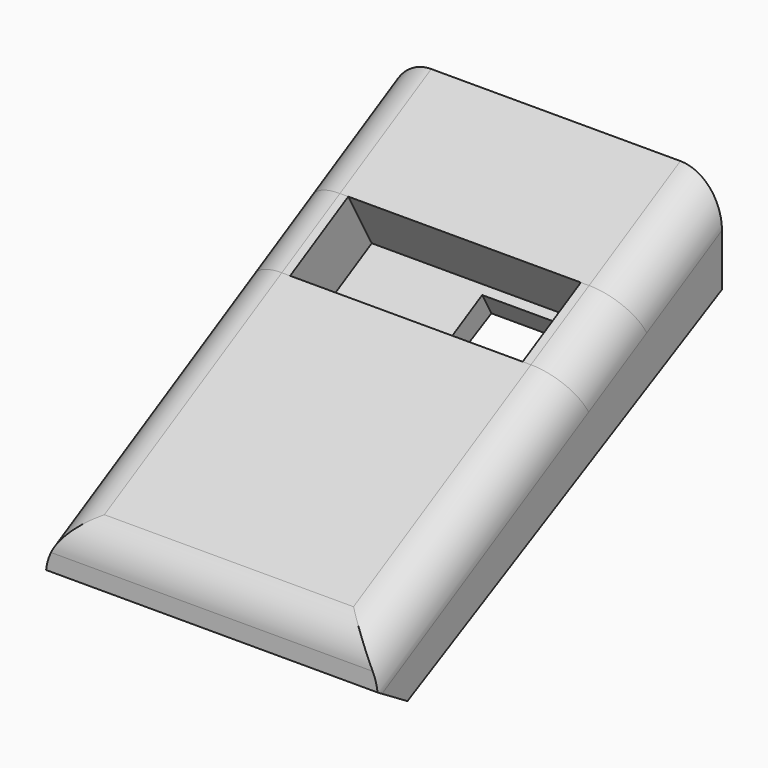
from build123d import *

# Parameters (mm, degrees)
F1_DEPTH = 40
F2_W     = 6
F2_H     = 7.3
F3_DEPTH = 10
F4_W     = 10.5
F4_H     = 8
F5_DEPTH = 25
F6_R     = 1.75
F7_DEPTH = 3
F8_R     = 5
F9_SIZE  = 5


with BuildPart() as f1:
    # F0 (on Right) → F1 (new body)
    with BuildSketch(Plane.YZ):
        Polygon((15.7016541125, 5.8919606872), (15.7016541125, 17.8919606872), (1.959085995, 10.2806947738), (5.4959338209, 3.8947173658), (-3.2519804366, -0.9502796561), (-6.7888282626, 5.435697752), (-36.0735021532, -10.7835007459), (-36.0735021532, -20.7835007459), align=None)
    extrude(amount=F1_DEPTH)

    # F2 (on face) → F3 (join, through all)
    with BuildSketch(Plane(origin=(0, 5.8565406788, 3.2436214293), x_dir=(1, 0, 0), z_dir=(0, -0.8747914258, -0.4844997022))):
        with Locations((3, 4.3942870579)):
            Rectangle(F2_W, F2_H)
        with Locations((37, 4.3942870579)):
            Rectangle(F2_W, F2_H)
    extrude(amount=F3_DEPTH)

    # F4 (on face) → F5 (cut)
    with BuildSketch(Plane(origin=(0, -0.3606068579, 0.6510959365), x_dir=(1, 0, 0), z_dir=(0, -0.4844997022, 0.8747914258))):
        with Locations((25.3092581406, 1.6064377211)):
            Rectangle(F4_W, F4_H)
    extrude(amount=-F5_DEPTH, mode=Mode.SUBTRACT)

    # F6 (on face) → F7 (join)
    with BuildSketch(Plane(origin=(0, 0.8948185727, -1.7367786325), x_dir=(1, 0, 0), z_dir=(0, 0.4580028747, -0.8889507111))):
        with Locations((35, -6.656531521)):
            Circle(F6_R)
        with Locations((5, -6.656531521)):
            Circle(F6_R)
        with Locations((35, 13.343468479)):
            Circle(F6_R)
        with Locations((5, 13.343468479)):
            Circle(F6_R)
    extrude(amount=F7_DEPTH)

    # F8
    f8_edges = [f1.edges().sort_by_distance(p)[0] for p in [
        (20, -36.073502, -10.783501),
        (40, -10.185924, 3.55423),
        (0, -10.185924, 3.55423),
    ]]
    fillet(f8_edges, radius=F8_R)

    # F9
    f9_edges = [f1.edges().sort_by_distance(p)[0] for p in [
        (20, -36.073502, -20.783501),
    ]]
    chamfer(f9_edges, length=F9_SIZE)


solid = f1.part
